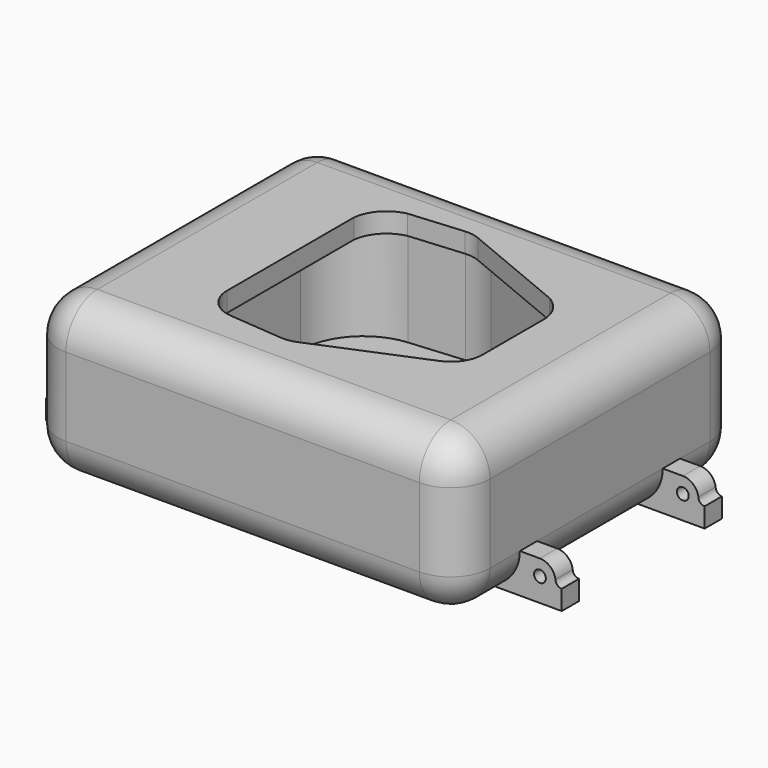
from build123d import *

# Parameters (mm, degrees)
F0_W              = 55
F0_H              = 45
F1_DEPTH          = 20
F5_DEPTH          = 17.5
F7_DEPTH          = 2.5
F9_R              = 5
F10_F1_R          = 5
F10_F2_R          = 5
F11_T1_DEPTH      = 35
F11_T3_DEPTH      = 62.5
F11_S7_W          = 5
F11_S7_H          = 5
F11_T8_DEPTH      = 5
F11_T12_ANGLE     = 90
F12_R             = 5
F15_R             = 0.75
F16_DEPTH         = 2.75
F16_COPIES2_COUNT = 2


# Not quite as in the source:
# - a fillet or chamfer that OpenCascade refuses, or shapes differently, is made with other operations: its cross-section is extruded or revolved along the edge and cut away or added
# - a feature of the source that left no trace in its solid (it failed there, or was rolled back) is left out
# - a pattern or mirror of a feature is missing from the dataset's text; its kind, count and spacing are read off the source's solid


with BuildPart() as f1:
    # F0 (on Top) → F1 (new body)
    with BuildSketch(Plane.XY):
        Rectangle(F0_W, F0_H)
    extrude(amount=F1_DEPTH)

    # F4 (on face) → F5 (cut)
    with BuildSketch(Plane.XY.offset(20)):
        with BuildLine():
            Line((-19.5686819828, 11.1526907945), (-19.5686819828, 1.0604560375))
            Line((-19.5686819828, 1.0604560375), (-19.5686819828, -9.0317787194))
            ThreePointArc((-19.5686819828, -9.0317787194), (-17.4612029419, -14.4427117948), (-12.2491327961, -17.0027878582))
            Line((-12.2491327961, -17.0027878582), (-5.4155437946, -17.5861419999))
            ThreePointArc((-5.4155437946, -17.5861419999), (-3.5037525417, -17.5198024128), (-1.6623660017, -17.0014952208))
            Line((-1.6623660017, -17.0014952208), (11.9654898342, -11.3323067543))
            ThreePointArc((11.9654898342, -11.3323067543), (15.5479043196, -8.3854367171), (16.8927628547, -3.9459443945))
            Line((16.8927628547, -3.9459443945), (16.8927628547, 1.0604560375))
            Line((16.8927628547, 1.0604560375), (16.8927628547, 6.0668564696))
            ThreePointArc((16.8927628547, 6.0668564696), (15.5479043196, 10.5063487921), (11.9654898342, 13.4532188293))
            Line((11.9654898342, 13.4532188293), (-1.6623660017, 19.1224072959))
            ThreePointArc((-1.6623660017, 19.1224072959), (-3.5037525417, 19.6407144879), (-5.4155437946, 19.7070540749))
            Line((-5.4155437946, 19.7070540749), (-12.2491327961, 19.1236999333))
            ThreePointArc((-12.2491327961, 19.1236999333), (-17.4612029419, 16.5636238699), (-19.5686819828, 11.1526907945))
        make_face()
    extrude(amount=-F5_DEPTH, mode=Mode.SUBTRACT)

    # F6 (on face) → F7 (join)
    with BuildSketch(Plane.XY.offset(20)):
        with BuildLine():
            ThreePointArc((-12.2491327961, 19.1236999333), (-17.4612029419, 16.5636238699), (-19.5686819828, 11.1526907945))
            Line((-19.5686819828, 11.1526907945), (-19.5686819828, -9.0317787194))
            ThreePointArc((-19.5686819828, -9.0317787194), (-17.4612029419, -14.4427117948), (-12.2491327961, -17.0027878582))
            Line((-12.2491327961, -17.0027878582), (-11.2008683554, -17.0922736911))
            Line((-11.2008683554, -17.0922736911), (-5.4155437946, -17.5861419999))
            ThreePointArc((-5.4155437946, -17.5861419999), (-3.5037525417, -17.5198024128), (-1.6623660017, -17.0014952208))
            Line((-1.6623660017, -17.0014952208), (11.9654898342, -11.3323067543))
            ThreePointArc((11.9654898342, -11.3323067543), (15.5479043196, -8.3854367171), (16.8927628547, -3.9459443945))
            Line((16.8927628547, -3.9459443945), (16.8927628547, 6.0668564696))
            ThreePointArc((16.8927628547, 6.0668564696), (15.5479043196, 10.5063487921), (11.9654898342, 13.4532188293))
            Line((11.9654898342, 13.4532188293), (-1.6432446132, 19.1144527977))
            Line((-1.6432446132, 19.1144527977), (-1.6623660017, 19.1224072959))
            ThreePointArc((-1.6623660017, 19.1224072959), (-3.5037525417, 19.6407144879), (-5.4155437946, 19.7070540749))
            Line((-5.4155437946, 19.7070540749), (-12.2491327961, 19.1236999333))
        make_face()
        with BuildLine():
            Line((-12.2647350556, -9.6505587512), (-12.2647350556, 0.4416760057))
            Line((-12.2647350556, 0.4416760057), (-12.2647350556, 10.5339107627))
            ThreePointArc((-12.2647350556, 10.5339107627), (-11.0828219735, 13.1216791931), (-8.6049604623, 14.5194153321))
            Line((-8.6049604623, 14.5194153321), (-1.7713714607, 15.1027694737))
            ThreePointArc((-1.7713714607, 15.1027694737), (-0.8154758343, 15.0695996802), (0.1052174357, 14.8104460842))
            Line((0.1052174357, 14.8104460842), (13.7330732716, 9.1412576176))
            ThreePointArc((13.7330732716, 9.1412576176), (15.4399139751, 7.6115436145), (16.1967097819, 5.4480764378))
            Line((16.1967097819, 5.4480764378), (16.1967097819, 0.4416760057))
            Line((16.1967097819, 0.4416760057), (16.1967097819, -4.5647244263))
            ThreePointArc((16.1967097819, -4.5647244263), (15.5242805143, -6.7844705876), (13.7330732716, -8.2579056062))
            Line((13.7330732716, -8.2579056062), (0.1052174357, -13.9270940728))
            ThreePointArc((0.1052174357, -13.9270940728), (-0.8154758343, -14.1862476688), (-1.7713714607, -14.2194174623))
            Line((-1.7713714607, -14.2194174623), (-8.6049604623, -13.6360633206))
            ThreePointArc((-8.6049604623, -13.6360633206), (-11.2109955351, -12.3560252889), (-12.2647350556, -9.6505587512))
        make_face(mode=Mode.SUBTRACT)
    extrude(amount=-F7_DEPTH)

    # F9
    f9_edges = [f1.edges().sort_by_distance(p)[0] for p in [
        (-27.5, -22.5, 10),
        (0, -22.5, 20),
    ]]
    fillet(f9_edges, radius=F9_R)

    # F10: fillet of radius 5 on 2 edges, made by hand

    # F10_f1
    f10_f1_edges = [f1.edges().sort_by_distance(p)[0] for p in [
        (0, 22.5, 0),
    ]]
    fillet(f10_f1_edges, radius=F10_F1_R)

    # F10_f2
    f10_f2_edges = [f1.edges().sort_by_distance(p)[0] for p in [
        (-27.5, 22.5, 12.5),
    ]]
    fillet(f10_f2_edges, radius=F10_F2_R)

    # F11: fillet of radius 5 on 2 edges, made by hand

    # F11_s2 → F11_t1 (cut)
    with BuildSketch(Plane.XZ.offset(-17.5)):
        with BuildLine():
            ThreePointArc((-22.5, 20), (-26.0355339059, 18.5355339059), (-27.5, 15))
            Line((-27.5, 15), (-27.5, 20))
            Line((-27.5, 20), (-22.5, 20))
        make_face()
    extrude(amount=F11_T1_DEPTH, mode=Mode.SUBTRACT)

    # F11_s4 → F11_t3 (cut)
    with BuildSketch(Plane.YZ.offset(-22.5)):
        with BuildLine():
            ThreePointArc((22.5, 15), (21.0355339059, 18.5355339059), (17.5, 20))
            Line((17.5, 20), (22.5, 20))
            Line((22.5, 20), (22.5, 15))
        make_face()
    extrude(amount=F11_T3_DEPTH, mode=Mode.SUBTRACT)


with BuildPart() as f11_tool6:
    # F11_s7 → F11_t8 (new body)
    with BuildSketch(Plane.XY.offset(15)):
        with Locations((-25, -20)):
            Rectangle(F11_S7_W, F11_S7_H)
    extrude(amount=F11_T8_DEPTH)

    # F11_s9 → F11_t10 (revolve, cut)
    with BuildSketch(Plane(origin=(-22.5, -17.5, 15), x_dir=(0.7071067812, 0.7071067812, 0), z_dir=(0.7071067812, -0.7071067812, 0))):
        with BuildLine():
            ThreePointArc((0, -5), (5, 0), (0, 5))
            Line((0, 5), (0, -5))
        make_face()
    revolve(axis=Axis((-22.5, -17.5, 15), (0, 0, 1)), mode=Mode.SUBTRACT)


with BuildPart() as f1_1:
    add(f1.part)

    # F11_t5: cut F11_tool6
    add(f11_tool6.part, mode=Mode.SUBTRACT)

    # F11_s11 → F11_t12 (revolve, cut)
    with BuildSketch(Plane.YZ.offset(-22.5)):
        with BuildLine():
            ThreePointArc((17.5, 20), (21.0355339059, 18.5355339059), (22.5, 15))
            Line((22.5, 15), (22.5, 20))
            Line((22.5, 20), (17.5, 20))
        make_face()
    revolve(axis=Axis((-22.5, 17.5, 20), (0, 0, 1)), revolution_arc=F11_T12_ANGLE, mode=Mode.SUBTRACT)

    # F12
    f12_edges = [f1_1.edges().sort_by_distance(p)[0] for p in [
        (-22.5, -22.5, 10),
        (27.5, 21.035534, 1.464466),
        (27.5, 22.5, 10),
        (27.5, 21.035534, 18.535534),
        (27.5, 0, 20),
        (27.5, -21.035534, 18.535534),
        (27.5, -22.5, 10),
        (27.5, -21.035534, 1.464466),
    ]]
    fillet(f12_edges, radius=F12_R)

    # F15 (on offset) → F16 (join)
    with BuildSketch(Plane.XZ.offset(12.75)):
        with BuildLine():
            Line((30.0576982113, 5), (27.5, 5))
            ThreePointArc((27.5, 5), (26.0355339059, 1.4644660941), (22.5, 0))
            Line((22.5, 0), (32.8350702046, 0))
            Line((32.8350702046, 0), (32.8350702046, 2.5))
            ThreePointArc((32.8350702046, 2.5), (32.2693847797, 2.7343145751), (32.0350702046, 3.3))
            ThreePointArc((32.0350702046, 3.3), (31.3615386923, 4.5165750888), (30.0576982113, 5))
        make_face()
        with Locations((30.0576982113, 3)):
            Circle(F15_R, mode=Mode.SUBTRACT)
    f16 = extrude(amount=-F16_DEPTH)

    # F16_copies: F16 across plane
    add(f16.mirror(Plane(origin=(0, 0, 0), x_dir=(0, 0, -1), z_dir=(-1, 0, 0))))

    # F16_copies1: F16 across plane
    add(f16.mirror(Plane.ZX))

    # F16_copies2: F16 ×2 about axis
    f16_copies2_axis = Axis((0, 0, 0), (0, 0, 1))
    for i in range(1, F16_COPIES2_COUNT):
        add(f16.rotate(f16_copies2_axis, i * 360 / F16_COPIES2_COUNT))


solid = f1_1.part
